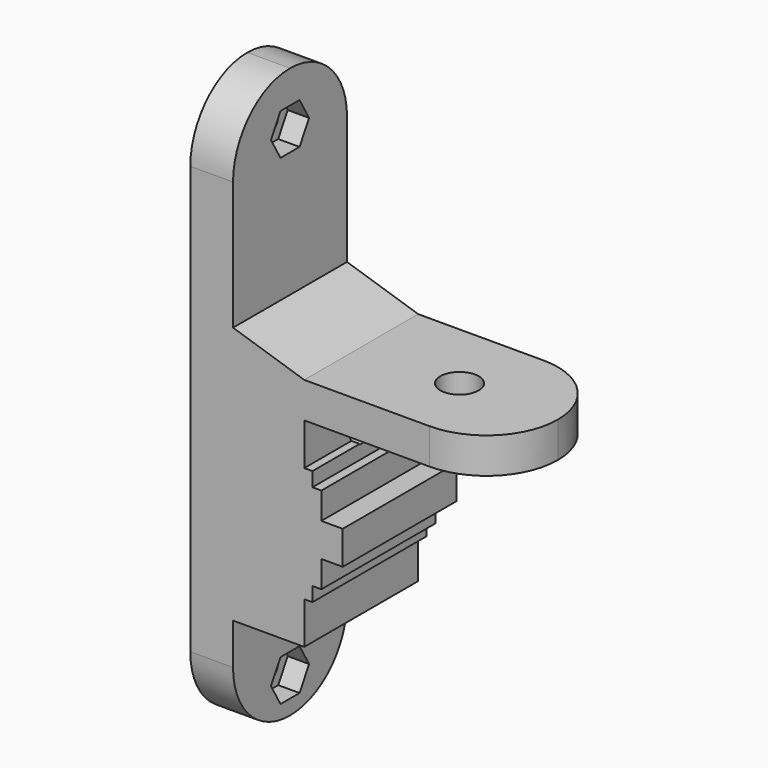
from build123d import *

# Parameters (mm, degrees)
F1_DEPTH       = 20
F2_R           = 2.7
F3_DEPTH       = 5
F4_R           = 1.7
F5_DEPTH       = 16.001
F6_R           = 1.7
F7_R           = 1.7
F9_DEPTH       = 3
F8_R           = 1.7
F10_DEPTH      = 5.4
F10_DEPTH_BACK = 13
F11_R          = 9.99999


# Not quite as in the source:
# - a fillet or chamfer is up to 0.001 mm smaller than in the source, because OpenCascade refuses the exact size


with BuildPart() as f1:
    # F0 (on Front) → F1 (new body)
    with BuildSketch(Plane.XZ):
        Polygon((16, 8.8), (6, 12), (6, 40), (0, 40), (0, -40), (6, -40), (6, -24.2), (16, -24.2), (16, -18.3), (17.15, -18.3), (17.15, -16.3), (18.4, -16.3), (18.4, -12.55), (21.4, -12.55), (21.4, -7.85), (18.4, -7.85), (18.4, -4.1), (17.15, -4.1), (17.15, -2.1), (16, -2.1), (16, 3.8), (43.6, 3.8), (43.6, 8.8), align=None)
    extrude(amount=F1_DEPTH)

    # F2 (on face) → F3 (cut, through all)
    with BuildSketch(Plane(origin=(0, 0, 3.8), x_dir=(1, 0, 0), z_dir=(0, 0, -1))):
        with Locations((29.8, 10)):
            Circle(F2_R)
    extrude(amount=-F3_DEPTH, mode=Mode.SUBTRACT)

    # F4 (on face) → F5 (cut, through all)
    with BuildSketch(Plane(origin=(0, 0, 0), x_dir=(0, -1, 0), z_dir=(-1, 0, 0))):
        with Locations((10, 32.5)):
            Circle(F4_R)
        with Locations((10, 0.7)):
            Circle(F4_R)
        with Locations((10, -35)):
            Circle(F4_R)
    extrude(amount=-F5_DEPTH, mode=Mode.SUBTRACT)

    # F6 (on face) + F7 (on face) → F9 (cut)
    with BuildSketch(Plane.YZ.offset(6)):
        Polygon((-13.3486315613, 32.5), (-11.6743157806, 29.6), (-8.3256842194, 29.6), (-6.6513684387, 32.5), (-8.3256842194, 35.4), (-11.6743157806, 35.4), align=None)
        with Locations((-10, 32.5)):
            Circle(F6_R, mode=Mode.SUBTRACT)
        with Locations((-10, 32.5)):
            Circle(F6_R)
    with BuildSketch(Plane.YZ.offset(6)):
        Polygon((-8.3256842194, -37.8999999998), (-6.6513684387, -34.9999999998), (-8.3256842194, -32.0999999998), (-11.6743157806, -32.0999999998), (-13.3486315613, -34.9999999998), (-11.6743157806, -37.8999999998), align=None)
        with Locations((-10, -35)):
            Circle(F7_R, mode=Mode.SUBTRACT)
    extrude(amount=-F9_DEPTH, mode=Mode.SUBTRACT)

    # F8 (on face) → F10 (cut, two sides)
    with BuildSketch(Plane.YZ.offset(16)) as f10_sk:
        Polygon((-13.3486315613, 0.7), (-11.7320508076, -2.1), (-8.2679491924, -2.1), (-6.6513684387, 0.7), (-8.3256842194, 3.6), (-11.6743157806, 3.6), align=None)
        with Locations((-10, 0.7)):
            Circle(F8_R, mode=Mode.SUBTRACT)
        Polygon((-11.7320508076, -2.1), (-11.6743157806, -2.2), (-8.3256842194, -2.2), (-8.2679491924, -2.1), align=None)
    extrude(amount=F10_DEPTH, mode=Mode.SUBTRACT)
    extrude(f10_sk.sketch, amount=-F10_DEPTH_BACK, mode=Mode.SUBTRACT)

    # F11 (radius 10 in the source; OpenCascade refuses exactly that, so slightly less here)
    f11_edges = [f1.edges().sort_by_distance(p)[0] for p in [
        (3, -20, 40),
        (3, 0, 40),
        (3, -20, -40),
        (3, 0, -40),
        (43.6, 0, 6.3),
        (43.6, -20, 6.3),
    ]]
    fillet(f11_edges, radius=F11_R)


solid = f1.part
